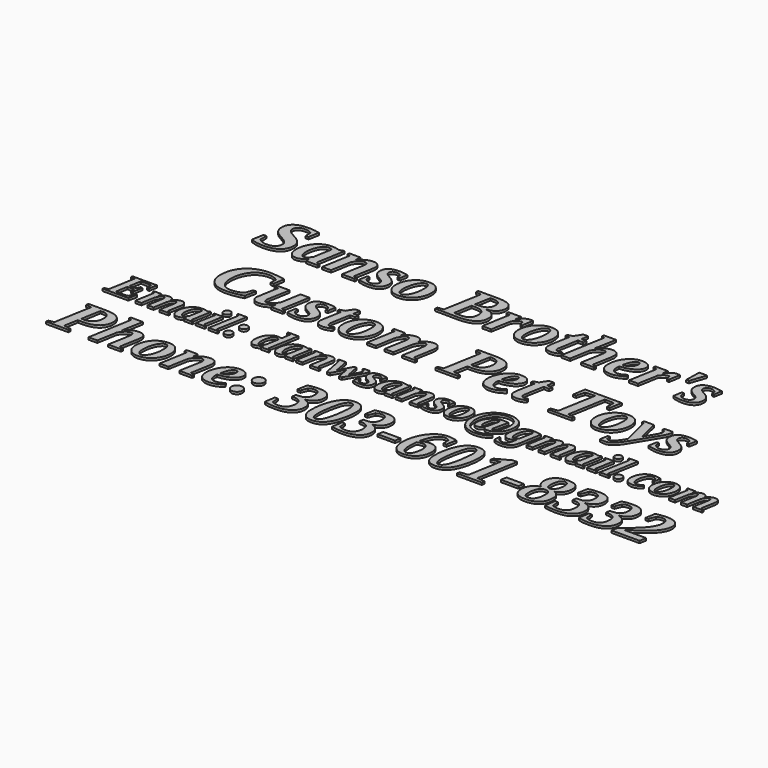
from build123d import *

# Parameters (mm, degrees)
F0_TEXT_SIZE   = 8.9951780656
F0_TEXT_SIZE_2 = 6.2498474158
F0_TEXT_SIZE_3 = 8.932777361
F1_DEPTH       = 0.3


# Not quite as in the source:
# - Text() gives the source's letters only with a copy of the font that has no kerning and outlines rounded to 1/6400 em; it was checked with that copy


with BuildPart() as f1:
    # F0 (on Top) → F1 (new body)
    with BuildSketch(Plane.XY):
        with Locations((-51.5627177954, -61.7443503611)):
            Text("Sanso Brother's", F0_TEXT_SIZE, font='Tinos', font_style=FontStyle.BOLDITALIC, text_align=(TextAlign.LEFT, TextAlign.BOTTOM))
        with Locations((-49.313923279, -72.0888051365)):
            Text('Custom Pet Toys', F0_TEXT_SIZE, font='Tinos', font_style=FontStyle.BOLDITALIC, text_align=(TextAlign.LEFT, TextAlign.BOTTOM))
        with Locations((-56.5627177954, -79.7677122933)):
            Text('Email: danwsanso@gmail.com', F0_TEXT_SIZE_2, font='Tinos', font_style=FontStyle.BOLDITALIC, text_align=(TextAlign.LEFT, TextAlign.BOTTOM))
        with Locations((-56.5627177954, -89.1994218538)):
            Text('Phone: 303-601-8332', F0_TEXT_SIZE_3, font='Tinos', font_style=FontStyle.BOLDITALIC, text_align=(TextAlign.LEFT, TextAlign.BOTTOM))
    extrude(amount=F1_DEPTH)


solid = f1.part
